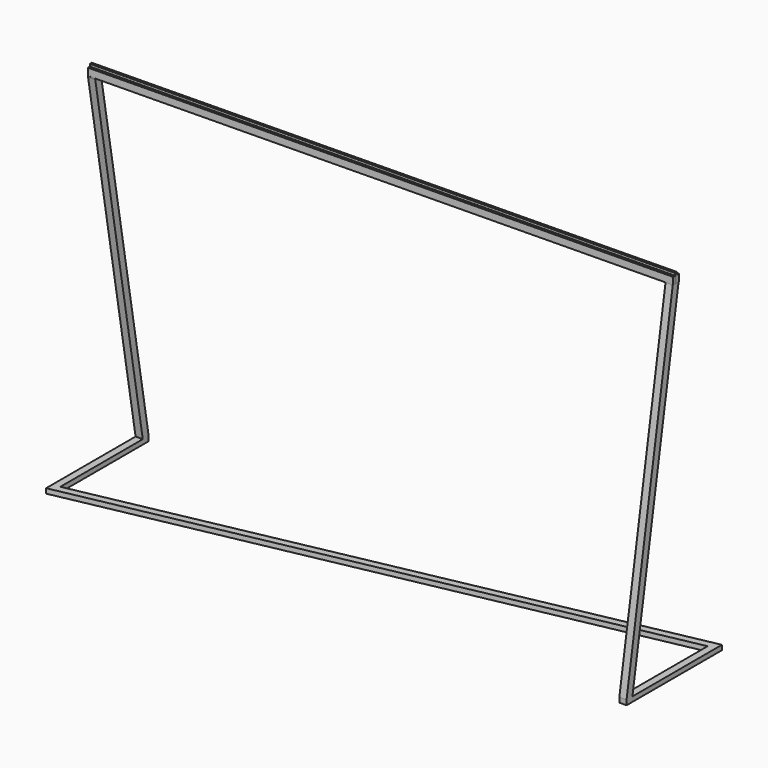
from build123d import *

# Parameters (mm, degrees)
F1_DEPTH = 25.4
F3_DEPTH = 38.1
F5_DEPTH = 38.1
F7_DEPTH = 38.1
F9_DEPTH = 12.7


# Not quite as in the source:
# - ends of sketch curves that miss each other by under 0.0002 mm in the source are joined


with BuildPart() as f1:
    # F0 (on Top) → F1 (new body)
    with BuildSketch(Plane.XY):
        Polygon((1524, -304.8), (1524, 324.2272643468), (-3.7360123744, 18.6800618719), (-3.0765473876, 15.3827369381), (179.8806457879, 16.5488648108), (1485.9, 277.7527356532), (1485.9, -9.5795955801), (1485.9, -304.8), align=None)
        Polygon((-1485.941186152, 124.6566928906), (-1485.9, 124.6078212585), (-1485.9, 183.7307214737), align=None)
        Polygon((179.8806457879, 16.5488648108), (-3.0765473876, 15.3827369381), (-20.7870508093, 15.2698541849), (-198.7212794918, -20.3169915516), (1.9464171055, -19.0379809257), align=None)
        Polygon((-3.0765473876, 15.3827369381), (-3.7360123744, 18.6800618719), (-20.7870508093, 15.2698541849), align=None)
        Polygon((1.9464171055, -19.0379809257), (-198.7212794918, -20.3169915516), (-1485.9, -277.7527356532), (-1485.9, 124.6078212585), (-1485.941186152, 124.6566928906), (-1485.9, 183.7307214737), (-1485.9, 304.8), (-1524, 304.8), (-1524, -324.2272643468), align=None)
    extrude(amount=F1_DEPTH)

    # F2 (on face) → F3 (join)
    with BuildSketch(Plane.YZ.offset(1524)):
        Polygon((-266.1596539356, 25.4), (0, 1600.1779524521), (0, 1828.8), (-304.8, 25.4), align=None)
        Polygon((0, 1828.8), (0, 1600.1779524521), (37.5672101274, 1822.4506123728), align=None)
        Polygon((38.6403460644, 1828.8), (0, 1828.8), (37.5672101274, 1822.4506123728), align=None)
    extrude(amount=-F3_DEPTH)

    # F4 (on face) → F5 (join)
    with BuildSketch(Plane(origin=(-1524, 0, 0), x_dir=(0, -1, 0), z_dir=(-1, 0, 0))):
        Polygon((9.7136321734, 1828.8), (9.7136321734, 1607.03972256), (47.2471081512, 1822.2541477998), align=None)
        Polygon((48.3887072147, 1828.8), (9.7136321734, 1828.8), (47.2471081512, 1822.2541477998), align=None)
        Polygon((-266.1249249587, 25.4), (9.7136321734, 1607.03972256), (9.7136321734, 1828.8), (-304.8, 25.4), align=None)
    extrude(amount=-F5_DEPTH)

    # F6 (on face) → F7 (join)
    with BuildSketch(Plane.XY.offset(1828.8)):
        Polygon((-1524, -29.0511696941), (-1524, -48.3887072147), (1526.0369777679, 0), (1526.0369777679, 12.9867385989), (-1523.899270198, -35.4003705418), align=None)
        Polygon((-1524.1007298046, -22.7019686808), (-1524, -29.0511696941), (-1524, -22.7003706067), align=None)
        Polygon((-1524, -22.7003706067), (-1524, -29.0511696941), (-1523.899270198, -35.4003705418), (1526.0369777679, 12.9867385989), (1526.0369777679, 19.3375375207), (1525.9362479633, 25.6867385339), align=None)
        Polygon((1526.0369777679, 19.3375375207), (1526.0369777679, 12.9867385989), (1526.1377075699, 12.9883366729), align=None)
        Polygon((-1524, -9.7136321734), (-1524, -22.7003706067), (1525.9362479633, 25.6867385339), (1526.0369777679, 19.3375375207), (1526.0369777679, 38.6750750413), align=None)
    extrude(amount=F7_DEPTH)

    # F8 (on face) → F9 (join)
    with BuildSketch(Plane.XY.offset(1866.9)):
        Polygon((1526.0369777679, 12.9867385989), (1525.9362479641, 25.6867384858), (-1524.1007298039, -22.701968729), (-1523.8992701954, -35.4003707073), align=None)
    extrude(amount=F9_DEPTH)


solid = f1.part
